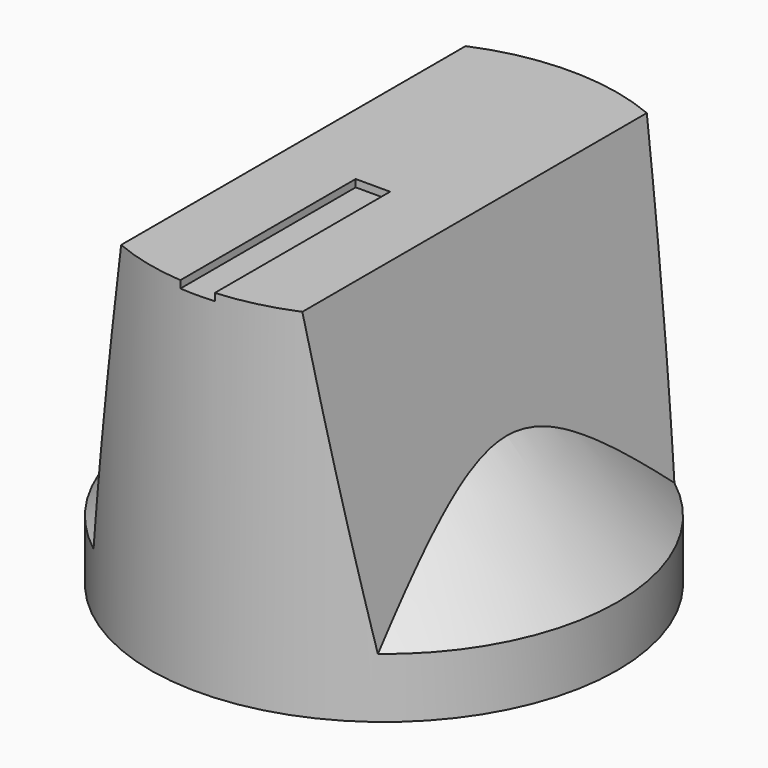
from build123d import *

# Parameters (mm, degrees)
F0_R     = 9.5
F1_DEPTH = 14.5
F2_R     = 3.15
F3_DEPTH = 13
F5_DEPTH = 12.5
F6_SIZE  = 4.49999
F7_W     = 1.4
F7_H     = 9.2790693743
F8_DEPTH = 0.3


# Not quite as in the source:
# - a fillet or chamfer is up to 0.001 mm smaller than in the source, because OpenCascade refuses the exact size


with BuildPart() as f1:
    # F0 (on Top) → F1 (new body)
    with BuildSketch(Plane.XY):
        Circle(F0_R)
    extrude(amount=F1_DEPTH)

    # F2 (on face) → F3 (cut)
    with BuildSketch(Plane(origin=(0, 0, 0), x_dir=(1, 0, 0), z_dir=(0, 0, -1))):
        Circle(F2_R)
    extrude(amount=-F3_DEPTH, mode=Mode.SUBTRACT)

    # F4 (on Front) → F5 (cut, symmetric)
    with BuildSketch(Plane.XZ):
        Polygon((5.0005883317, 16.3299063618), (3.68460026, 14.5), (5, 6.9363636364), (9.7186830602, 6.9363636364), (12.480460446, 14.9852110131), align=None)
        Polygon((-5, 6.9363636364), (-3.68460026, 14.5), (-5.0005883317, 16.3299063618), (-12.480460446, 14.9852110131), (-9.7186830602, 6.9363636364), align=None)
    extrude(amount=F5_DEPTH, both=True, mode=Mode.SUBTRACT)

    # F6 (size 4.5 in the source; OpenCascade refuses exactly that, so slightly less here)
    f6_edges = [f1.edges().sort_by_distance(p)[0] for p in [
        (8.299096, -4.623311, 6.936364),
        (8.299096, 4.623311, 6.936364),
        (-9.5, 0, 6.936364),
    ]]
    chamfer(f6_edges, length=F6_SIZE)

    # F7 (on face) → F8 (cut)
    with BuildSketch(Plane.XY.offset(14.5)):
        with Locations((0, -5.2029067301)):
            Rectangle(F7_W, F7_H)
    extrude(amount=-F8_DEPTH, mode=Mode.SUBTRACT)


solid = f1.part
